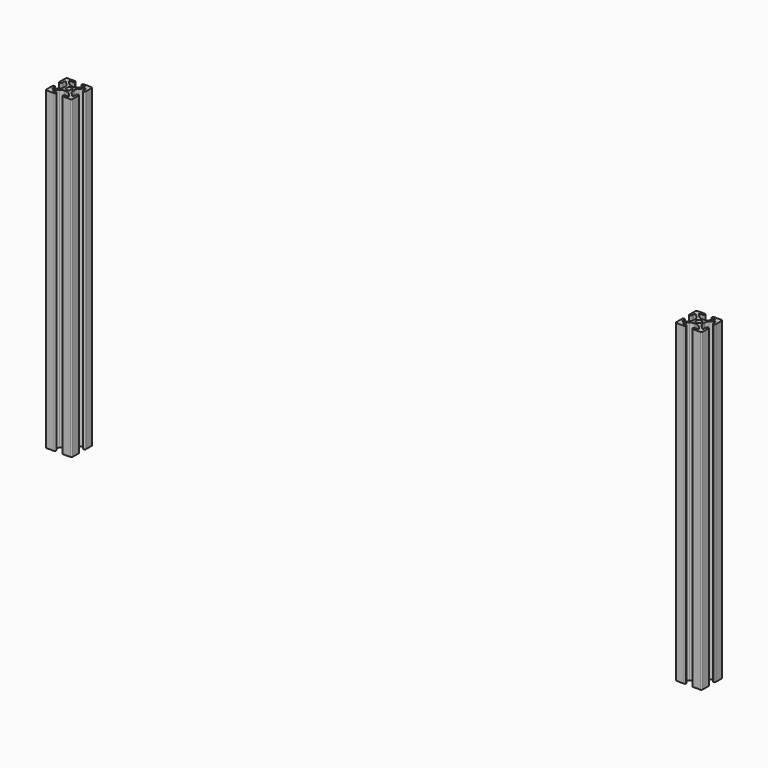
from build123d import *

# Parameters (mm, degrees)
F0_R     = 2.6035
F1_DEPTH = 304.8
F2_R     = 1.18109
F3_R     = 5.08
F4_R     = 0.762
F5_R     = 1.27


# Not quite as in the source:
# - a fillet or chamfer is up to 0.001 mm smaller than in the source, because OpenCascade refuses the exact size


with BuildPart() as f1:
    # F0 (on Top) → F1 (new body)
    with BuildSketch(Plane.XY):
        Polygon((12.7, 3.2385), (12.7, 12.7), (3.2385, 12.7), (3.2385, 10.3378), (8.7752354349, 10.3378), (2.9459354349, 4.5085), (-2.9459354349, 4.5085), (-8.7752354349, 10.3378), (-3.2385, 10.3378), (-3.2385, 12.7), (-12.7, 12.7), (-12.7, 3.2385), (-10.3378, 3.2385), (-10.3378, 8.7752354349), (-4.5085, 2.9459354349), (-4.5085, -2.9459354349), (-10.3378, -8.7752354349), (-10.3378, -3.2385), (-12.7, -3.2385), (-12.7, -12.7), (-3.2385, -12.7), (-3.2385, -10.3378), (-8.7752354349, -10.3378), (-2.9459354349, -4.5085), (2.9459354349, -4.5085), (8.7752354349, -10.3378), (3.2385, -10.3378), (3.2385, -12.7), (12.7, -12.7), (12.7, -3.2385), (10.3378, -3.2385), (10.3378, -8.7752354349), (4.5085, -2.9459354349), (4.5085, 2.9459354349), (10.3378, 8.7752354349), (10.3378, 3.2385), align=None)
        Circle(F0_R, mode=Mode.SUBTRACT)
    extrude(amount=F1_DEPTH)

    # F2 (radius 1.1811 in the source; OpenCascade refuses exactly that, so slightly less here)
    f2_edges = [f1.edges().sort_by_distance(p)[0] for p in [
        (3.2385, 12.7, 152.4),
        (3.2385, 10.3378, 152.4),
        (-3.2385, 12.7, 152.4),
        (-12.7, 3.2385, 152.4),
        (-3.2385, 10.3378, 152.4),
        (-10.3378, 3.2385, 152.4),
        (12.7, 3.2385, 152.4),
        (10.3378, 3.2385, 152.4),
        (12.7, -3.2385, 152.4),
        (10.3378, -3.2385, 152.4),
        (3.2385, -10.3378, 152.4),
        (-3.2385, -10.3378, 152.4),
        (-10.3378, -3.2385, 152.4),
        (-12.7, -3.2385, 152.4),
        (-3.2385, -12.7, 152.4),
        (3.2385, -12.7, 152.4),
    ]]
    fillet(f2_edges, radius=F2_R)

    # F3
    f3_edges = [f1.edges().sort_by_distance(p)[0] for p in [
        (2.945935, 4.5085, 152.4),
        (-2.945935, 4.5085, 152.4),
        (4.5085, -2.945935, 152.4),
        (4.5085, 2.945935, 152.4),
        (2.945935, -4.5085, 152.4),
        (-2.945935, -4.5085, 152.4),
        (-4.5085, -2.945935, 152.4),
        (-4.5085, 2.945935, 152.4),
    ]]
    fillet(f3_edges, radius=F3_R)

    # F4
    f4_edges = [f1.edges().sort_by_distance(p)[0] for p in [
        (8.775235, 10.3378, 152.4),
        (-8.775235, 10.3378, 152.4),
        (-10.3378, 8.775235, 152.4),
        (-10.3378, -8.775235, 152.4),
        (-8.775235, -10.3378, 152.4),
        (8.775235, -10.3378, 152.4),
        (10.3378, -8.775235, 152.4),
        (10.3378, 8.775235, 152.4),
    ]]
    fillet(f4_edges, radius=F4_R)

    # F5
    f5_edges = [f1.edges().sort_by_distance(p)[0] for p in [
        (-12.7, -12.7, 152.4),
        (12.7, -12.7, 152.4),
        (12.7, 12.7, 152.4),
        (-12.7, 12.7, 152.4),
    ]]
    fillet(f5_edges, radius=F5_R)


with BuildPart() as f6_1:
    # F6: copy of F1
    add(f1.part.moved(Location((609.6, 0, 0))))


solid = Compound([f1.part, f6_1.part])
